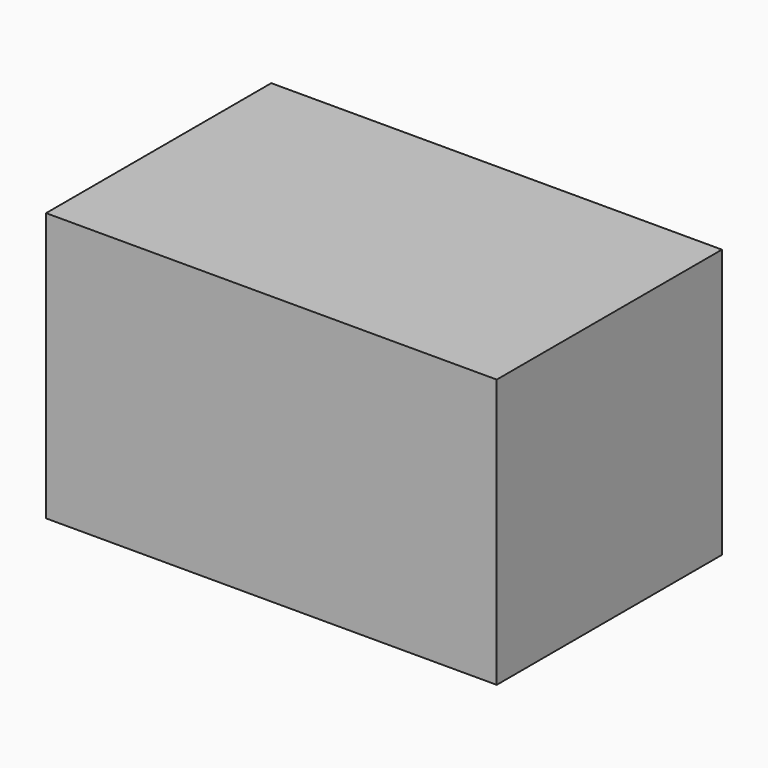
from build123d import *

# Parameters (mm, degrees)
F0_W     = 60.3929003701
F0_H     = 33.9642912149
F1_DEPTH = 35.814
F2_T     = 2.54


with BuildPart() as f1:
    # F0 (on Front) → F1 (new body)
    with BuildSketch(Plane.XZ):
        with Locations((-40.0745426305, 29.1485004127)):
            Rectangle(F0_W, F0_H)
    extrude(amount=F1_DEPTH)

    # F2 (hollow, outwards: the wall grows on the outside; the body as it was is the cavity)
    f2_inside = f1.part
    offset(amount=F2_T, kind=Kind.INTERSECTION)
    add(f2_inside, mode=Mode.SUBTRACT)


solid = f1.part
